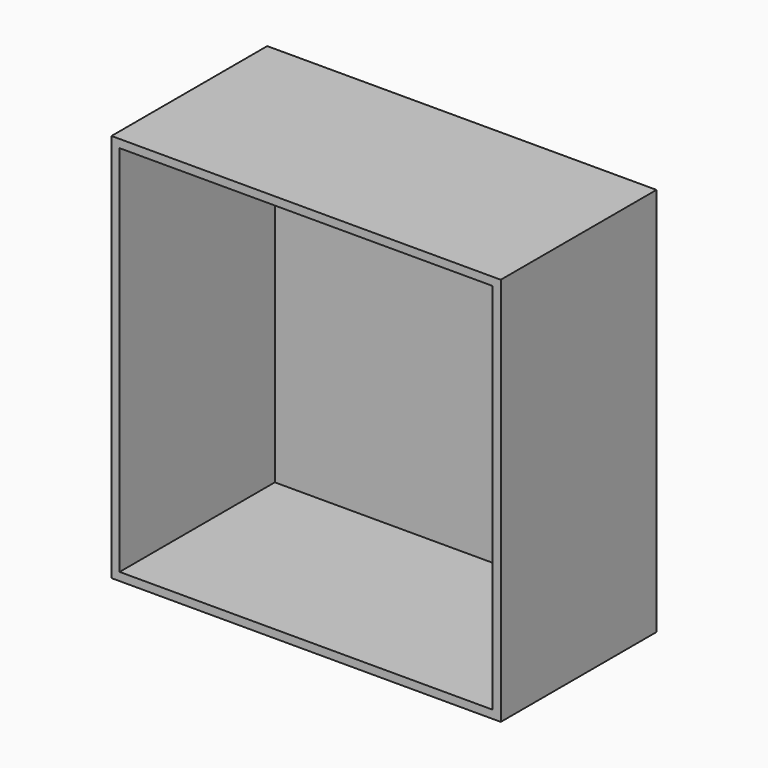
from build123d import *

# Parameters (mm, degrees)
F0_W     = 120
F0_H     = 120
F1_DEPTH = 60
F2_W     = 115
F2_H     = 115
F3_DEPTH = 59.8


# Not quite as in the source:
# - the program builds the solid bodies; features that only make, move or delete a surface that nothing else refers to are left out


with BuildPart() as f1:
    # F0 (on Front) → F1 (new body)
    with BuildSketch(Plane.XZ):
        Rectangle(F0_W, F0_H)
    extrude(amount=-F1_DEPTH)

    # F2 (on Front) → F3 (cut)
    with BuildSketch(Plane.XZ):
        Rectangle(F2_W, F2_H)
    extrude(amount=-F3_DEPTH, mode=Mode.SUBTRACT)


solid = f1.part
